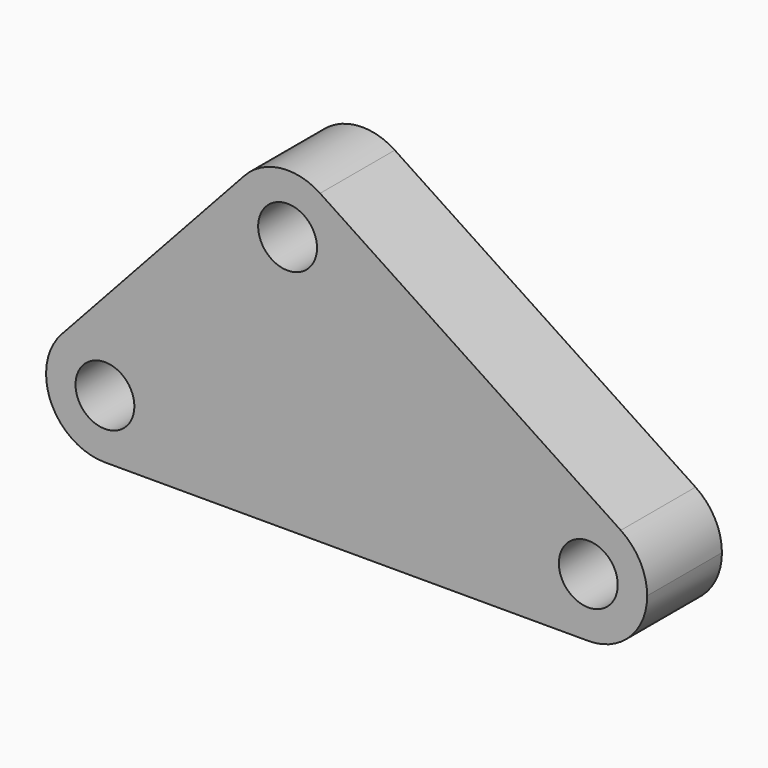
from build123d import *

# Parameters (mm, degrees)
F1_DEPTH = 12.7
F2_R     = 4
F3_DEPTH = 12.7


with BuildPart() as f1:
    # F0 (on Front) → F1 (new body)
    with BuildSketch(Plane.XZ):
        with BuildLine():
            Line((-35.8775282965, 24.0157592565), (-21.8738068975, 39.259964286))
            ThreePointArc((-21.8738068975, 39.259964286), (-24.4545549996, 44.812447626), (-22.3532208609, 50.5635107317))
            Line((-22.3532208609, 50.5635107317), (-47.1810747422, 23.536345293))
            ThreePointArc((-47.1810747422, 23.536345293), (-41.6285914022, 26.1170933952), (-35.8775282965, 24.0157592565))
        make_face()
        with BuildLine():
            Line((-21.8738068975, 39.259964286), (-16.4617406563, 45.1514444906))
            Line((-16.4617406563, 45.1514444906), (-9.7887372084, 40.7388460516))
            ThreePointArc((-9.7887372084, 40.7388460516), (-8.8006693349, 42.8475377633), (-8.4617406563, 45.1514444906))
            ThreePointArc((-8.4617406563, 45.1514444906), (-9.4154371037, 48.939531903), (-12.0491422174, 51.8244479385))
            ThreePointArc((-12.0491422174, 51.8244479385), (-17.4334728618, 53.0922087183), (-22.3532208609, 50.5635107317))
            ThreePointArc((-22.3532208609, 50.5635107317), (-24.4545549996, 44.812447626), (-21.8738068975, 39.259964286))
        make_face()
        with BuildLine():
            ThreePointArc((-9.7887372084, 40.7388460516), (-15.4900084509, 37.2106802628), (-21.8738068975, 39.259964286))
            Line((-21.8738068975, 39.259964286), (-35.8775282965, 24.0157592565))
            ThreePointArc((-35.8775282965, 24.0157592565), (-33.9650969463, 21.3416902838), (-33.2895945376, 18.1242790519))
            Line((-33.2895945376, 18.1242790519), (16.4104054624, 18.1242790519))
            ThreePointArc((16.4104054624, 18.1242790519), (16.749334141, 20.4281857792), (17.7374020144, 22.5368774909))
            Line((17.7374020144, 22.5368774909), (-9.7887372084, 40.7388460516))
        make_face()
        with BuildLine():
            Line((-9.7887372084, 40.7388460516), (-16.4617406563, 45.1514444906))
            Line((-16.4617406563, 45.1514444906), (-21.8738068975, 39.259964286))
            ThreePointArc((-21.8738068975, 39.259964286), (-15.4900084509, 37.2106802628), (-9.7887372084, 40.7388460516))
        make_face()
        with BuildLine():
            ThreePointArc((-8.4617406563, 45.1514444906), (-8.8006693349, 42.8475377633), (-9.7887372084, 40.7388460516))
            Line((-9.7887372084, 40.7388460516), (17.7374020144, 22.5368774909))
            ThreePointArc((17.7374020144, 22.5368774909), (22.8120577523, 25.9629833197), (28.8230039014, 24.7972824999))
            Line((28.8230039014, 24.7972824999), (-12.0491422174, 51.8244479385))
            ThreePointArc((-12.0491422174, 51.8244479385), (-9.4154371037, 48.939531903), (-8.4617406563, 45.1514444906))
        make_face()
        with BuildLine():
            ThreePointArc((28.8230039014, 24.7972824999), (22.8120577523, 25.9629833197), (17.7374020144, 22.5368774909))
            Line((17.7374020144, 22.5368774909), (24.4104054624, 18.1242790519))
            Line((24.4104054624, 18.1242790519), (16.4104054624, 18.1242790519))
            ThreePointArc((16.4104054624, 18.1242790519), (18.7535512129, 12.4674248024), (24.4104054624, 10.1242790519))
            ThreePointArc((24.4104054624, 10.1242790519), (30.0672597119, 12.4674248024), (32.4104054624, 18.1242790519))
            ThreePointArc((32.4104054624, 18.1242790519), (31.456709015, 21.9123664643), (28.8230039014, 24.7972824999))
        make_face()
        with BuildLine():
            Line((24.4104054624, 18.1242790519), (17.7374020144, 22.5368774909))
            ThreePointArc((17.7374020144, 22.5368774909), (16.749334141, 20.4281857792), (16.4104054624, 18.1242790519))
            Line((16.4104054624, 18.1242790519), (24.4104054624, 18.1242790519))
        make_face()
        with BuildLine():
            Line((16.4104054624, 18.1242790519), (-33.2895945376, 18.1242790519))
            ThreePointArc((-33.2895945376, 18.1242790519), (-35.6327402881, 12.4674248024), (-41.2895945376, 10.1242790519))
            Line((-41.2895945376, 10.1242790519), (24.4104054624, 10.1242790519))
            ThreePointArc((24.4104054624, 10.1242790519), (18.7535512129, 12.4674248024), (16.4104054624, 18.1242790519))
        make_face()
        with BuildLine():
            Line((-41.2895945376, 18.1242790519), (-35.8775282965, 24.0157592565))
            ThreePointArc((-35.8775282965, 24.0157592565), (-41.6285914022, 26.1170933952), (-47.1810747422, 23.536345293))
            ThreePointArc((-47.1810747422, 23.536345293), (-48.6140921289, 14.90686782), (-41.2895945376, 10.1242790519))
            ThreePointArc((-41.2895945376, 10.1242790519), (-35.6327402881, 12.4674248024), (-33.2895945376, 18.1242790519))
            Line((-33.2895945376, 18.1242790519), (-41.2895945376, 18.1242790519))
        make_face()
        with BuildLine():
            ThreePointArc((-33.2895945376, 18.1242790519), (-33.9650969463, 21.3416902838), (-35.8775282965, 24.0157592565))
            Line((-35.8775282965, 24.0157592565), (-41.2895945376, 18.1242790519))
            Line((-41.2895945376, 18.1242790519), (-33.2895945376, 18.1242790519))
        make_face()
    extrude(amount=F1_DEPTH)

    # F2 (on face) → F3 (cut, through all)
    with BuildSketch(Plane.XZ.offset(12.7)):
        with Locations((-16.4617406563, 45.1514444906)):
            Circle(F2_R)
        with Locations((-41.2895945376, 18.1242790519)):
            Circle(F2_R)
        with Locations((24.4104054624, 18.1242790519)):
            Circle(F2_R)
    extrude(amount=-F3_DEPTH, mode=Mode.SUBTRACT)


solid = f1.part
